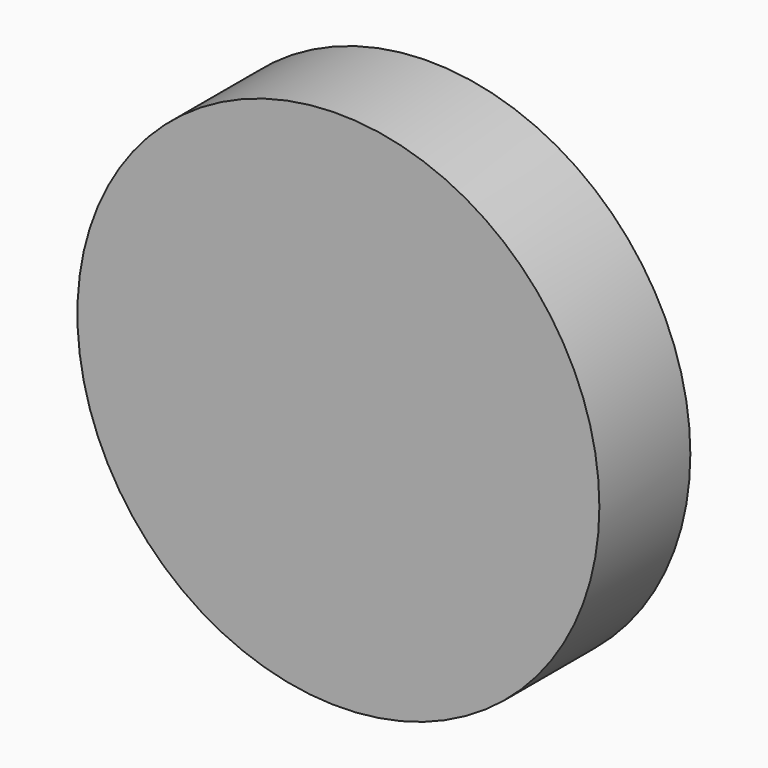
from build123d import *

# Parameters (mm, degrees)
F0_R     = 58.2968081569
F1_DEPTH = 25.4


# Not quite as in the source:
# - the program builds the solid bodies; features that only make, move or delete a surface that nothing else refers to are left out


with BuildPart() as f1:
    # F0 (on Front) → F1 (new body)
    with BuildSketch(Plane.XZ):
        Circle(F0_R)
    extrude(amount=F1_DEPTH)

    # F5: F1 across plane


with BuildPart() as f1_1:
    add(f1.part)
    add(f1.part.mirror(Plane.XY))


solid = f1_1.part
